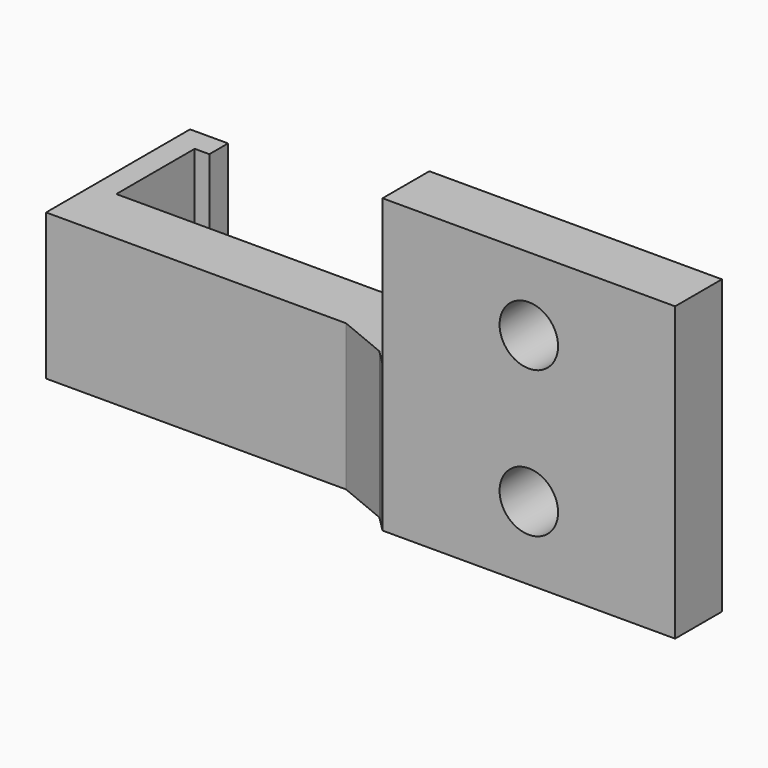
from build123d import *

# Parameters (mm, degrees)
F0_W        = 20
F0_H        = 2.5
F1_DEPTH    = 9.2
F2_DEPTH    = 10
F3_R        = 2
F4_DEPTH    = 25
F5_W        = 1
F5_H        = 6.7
F6_DEPTH    = 0.8
F7_T1_DEPTH = 10
F7_T6_DEPTH = 20.3706815716
F8_ANGLE    = 180


# Not quite as in the source:
# - a fillet or chamfer that OpenCascade refuses, or shapes differently, is made with other operations: its cross-section is extruded or revolved along the edge and cut away or added


with BuildPart() as f1:
    # F0 (on Top) → F1 (new body)
    with BuildSketch(Plane.XY):
        Polygon((-9.1, -3.35), (-10.1, -3.35), (-10.1, 3.35), (10.1, 3.35), (10.1, -3.35), (9.1, -3.35), (9.1, -4.95), (11.7, -4.95), (11.7, 3.35), (11.7, 7.35), (10.8, 7.35), (-11.7, 7.35), (-11.7, -4.95), (-9.1, -4.95), align=None)
        Polygon((13.3, 7.35), (11.7, 7.35), (11.7, 3.35), (13.3, 3.35), (13.3, 5.85), align=None)
        Polygon((13.3, 9.85), (10.8, 7.35), (11.7, 7.35), (13.3, 7.35), align=None)
        with Locations((23.3, 8.6)):
            Rectangle(F0_W, F0_H)
        Polygon((33.3, 7.35), (13.3, 7.35), (13.3, 5.85), (15.8, 5.85), (33.3, 5.85), align=None)
        Polygon((13.3, 5.85), (13.3, 3.35), (15.8, 5.85), align=None)
    extrude(amount=F1_DEPTH)

    # F0 (on Top) → F2 (join, symmetric)
    with BuildSketch(Plane.XY):
        Polygon((33.3, 7.35), (13.3, 7.35), (13.3, 5.85), (15.8, 5.85), (33.3, 5.85), align=None)
        with Locations((23.3, 8.6)):
            Rectangle(F0_W, F0_H)
    extrude(amount=F2_DEPTH, both=True)

    # F3 (on face) → F4 (cut)
    with BuildSketch(Plane.XZ.offset(-5.85)):
        with Locations((23.3, 5)):
            Circle(F3_R)
        with Locations((23.3, -5)):
            Circle(F3_R)
    extrude(amount=-F4_DEPTH, mode=Mode.SUBTRACT)

    # F5 (on face) → F6 (join, through all)
    with BuildSketch(Plane.XY.offset(9.2)):
        Polygon((-9.1, -4.95), (-9.1, -3.35), (-10.1, -3.35), (-10.1, 3.35), (-9.1, 3.35), (9.1, 3.35), (10.1, 3.35), (10.1, -3.35), (9.1, -3.35), (9.1, -4.95), (11.7, -4.95), (11.7, 3.35), (13.3, 3.35), (15.8, 5.85), (13.3, 5.85), (13.3, 9.85), (10.8, 7.35), (-11.7, 7.35), (-11.7, -4.95), align=None)
        with Locations((-9.6, 0)):
            Rectangle(F5_W, F5_H)
        with Locations((9.6, 0)):
            Rectangle(F5_W, F5_H)
    extrude(amount=F6_DEPTH)

    # F7: chamfer of 2 on 2 edges, made by hand

    # F7_s2 → F7_t1 (join)
    with BuildSketch(Plane.XY):
        Polygon((12.2142135624, 8.7642135624), (8.8, 7.35), (10.8, 7.35), align=None)
    extrude(amount=F7_T1_DEPTH)


with BuildPart() as f7_tool4:
    # F7_s5 → F7_t6 (new body)
    with BuildSketch(Plane.XY.offset(15.1853407858)):
        Polygon((11.3, 3.35), (14.7142135624, 4.7642135624), (13.3, 3.35), align=None)
    extrude(amount=-F7_T6_DEPTH)

    split(bisect_by=Plane.YZ.offset(11.7), keep=Keep.TOP)


with BuildPart() as f1_1:
    add(f1.part)

    # F7_t3: cut F7_tool4
    add(f7_tool4.part, mode=Mode.SUBTRACT)


with BuildPart() as f1_2:
    # F8: moved
    add(f1_1.part.rotate(Axis((24.55, 5.85, 10), (1, 0, 0)), F8_ANGLE))


solid = f1_2.part
